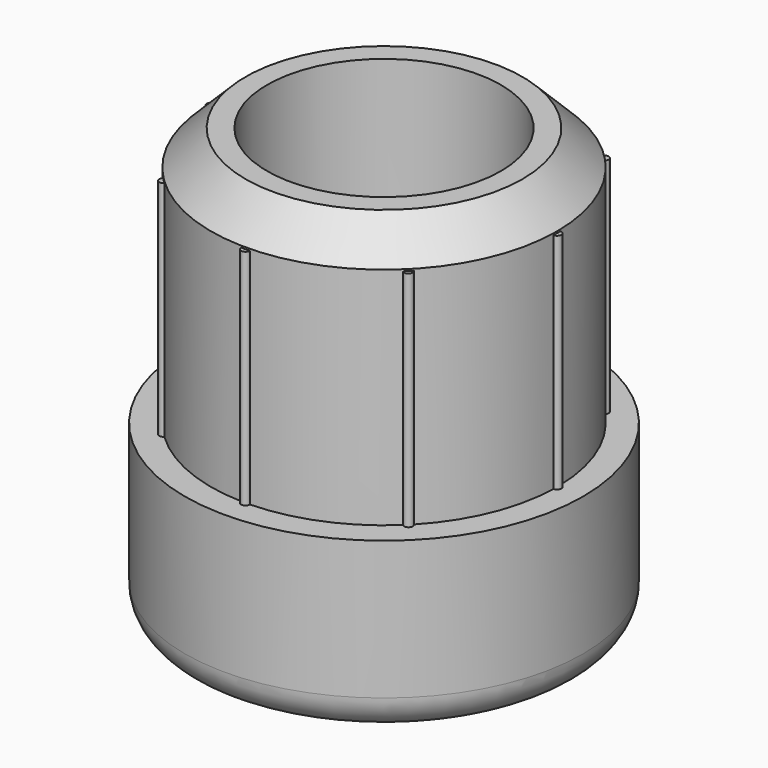
from build123d import *

# Parameters (mm, degrees)
F0_R          = 11.5
F1_DEPTH      = 10
F2_R          = 6.75
F3_DEPTH      = 6
F4_R          = 10
F4_R_2        = 6.75
F5_DEPTH      = 15
F6_R          = 2
F8_DEPTH      = 12.9
F9_SIZE       = 2
F10_TEXT_SIZE = 18.5950843103
F11_DEPTH     = 1


# Not quite as in the source:
# - Text() gives the source's letters only with a copy of the font that has no kerning and outlines rounded to 1/6400 em; it was checked with that copy


with BuildPart() as f1:
    # F0 (on Top) → F1 (new body)
    with BuildSketch(Plane.XY):
        Circle(F0_R)
    extrude(amount=F1_DEPTH)

    # F2 (on face) → F3 (cut)
    with BuildSketch(Plane.XY.offset(10)):
        Circle(F2_R)
    extrude(amount=-F3_DEPTH, mode=Mode.SUBTRACT)

    # F4 (on face) → F5 (join)
    with BuildSketch(Plane.XY.offset(10)):
        Circle(F4_R)
        Circle(F4_R_2, mode=Mode.SUBTRACT)
    extrude(amount=F5_DEPTH)

    # F6
    f6_edges = [f1.edges().sort_by_distance(p)[0] for p in [
        (-11.5, 0, 0),
    ]]
    fillet(f6_edges, radius=F6_R)

    # F7 (on face) → F8 (join)
    with BuildSketch(Plane.XY.offset(10)):
        with BuildLine():
            ThreePointArc((-0.25, 9.9968745116), (0, 10), (0.25, 9.9968745116))
            ThreePointArc((0.25, 9.9968745116), (0, 10.2500195366), (-0.25, 9.9968745116))
        make_face()
        with BuildLine():
            ThreePointArc((7.2456209873, 6.8920952191), (7.2478445072, 7.2478445072), (6.8920952191, 7.2456209873))
            ThreePointArc((6.8920952191, 7.2456209873), (7.0710678119, 7.0710678119), (7.2456209873, 6.8920952191))
        make_face()
        with BuildLine():
            ThreePointArc((9.9968745116, -0.25), (10.2500195366, 0), (9.9968745116, 0.25))
            ThreePointArc((9.9968745116, 0.25), (9.9992185974, 0.1250097683), (10, 0))
            ThreePointArc((10, 0), (9.9992185974, -0.1250097683), (9.9968745116, -0.25))
        make_face()
        with BuildLine():
            ThreePointArc((6.8920952191, -7.2456209873), (7.2478445072, -7.2478445072), (7.2456209873, -6.8920952191))
            ThreePointArc((7.2456209873, -6.8920952191), (7.0710678119, -7.0710678119), (6.8920952191, -7.2456209873))
        make_face()
        with BuildLine():
            ThreePointArc((-0.25, -9.9968745116), (0, -10.2500195366), (0.25, -9.9968745116))
            ThreePointArc((0.25, -9.9968745116), (0, -10), (-0.25, -9.9968745116))
        make_face()
        with BuildLine():
            ThreePointArc((-6.8920952191, -7.2456209873), (-7.0710678119, -7.0710678119), (-7.2456209873, -6.8920952191))
            ThreePointArc((-7.2456209873, -6.8920952191), (-7.2478445072, -7.2478445072), (-6.8920952191, -7.2456209873))
        make_face()
        with BuildLine():
            ThreePointArc((-9.9968745116, -0.25), (-10, 0), (-9.9968745116, 0.25))
            ThreePointArc((-9.9968745116, 0.25), (-10.2500195366, 0), (-9.9968745116, -0.25))
        make_face()
        with BuildLine():
            ThreePointArc((-7.2456209873, 6.8920952191), (-7.0710678119, 7.0710678119), (-6.8920952191, 7.2456209873))
            ThreePointArc((-6.8920952191, 7.2456209873), (-7.2478445072, 7.2478445072), (-7.2456209873, 6.8920952191))
        make_face()
    extrude(amount=F8_DEPTH)

    # F9
    f9_edges = [f1.edges().sort_by_distance(p)[0] for p in [
        (-10, 0, 25),
    ]]
    chamfer(f9_edges, length=F9_SIZE)

    # F10 (on face) → F11 (cut)
    with BuildSketch(Plane(origin=(0, 0, 0), x_dir=(1, 0, 0), z_dir=(0, 0, -1))):
        with Locations((-6.7407180625, -6.6942303517)):
            Text('R', F10_TEXT_SIZE, font='Open Sans', font_style=FontStyle.BOLD, text_align=(TextAlign.LEFT, TextAlign.BOTTOM))
    extrude(amount=-F11_DEPTH, mode=Mode.SUBTRACT)


solid = f1.part
